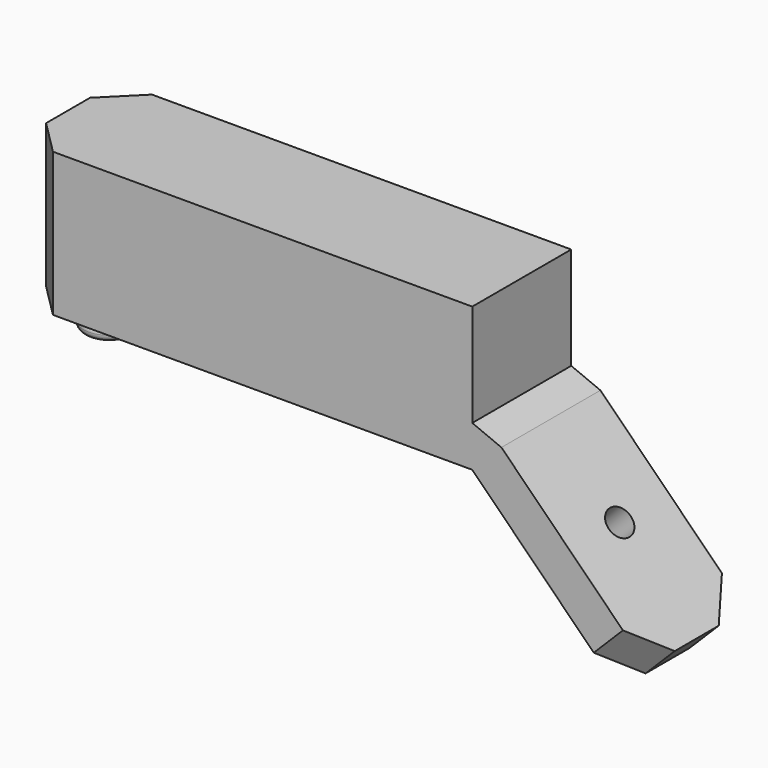
from build123d import *

# Parameters (mm, degrees)
F0_R      = 3.75
F1_DEPTH  = 2
F2_R      = 1
F3_DEPTH  = 3
F4_W      = 37.5
F4_H      = 18
F5_DEPTH  = 6
F7_DEPTH  = 18
F8_R      = 2
F9_DEPTH  = 37.8
F10_R     = 0.99999
F11_SIZE  = 5
F12_DEPTH = 14.9


# Not quite as in the source:
# - a fillet or chamfer is up to 0.001 mm smaller than in the source, because OpenCascade refuses the exact size


with BuildPart() as f1:
    # F0 (on Top) → F1 (new body)
    with BuildSketch(Plane.XY):
        Circle(F0_R)
    extrude(amount=F1_DEPTH)

    # F2 (on face) → F3 (join)
    with BuildSketch(Plane.XY.offset(2)):
        Circle(F2_R)
    extrude(amount=F3_DEPTH)

    # F4 (on face) → F5 (join)
    with BuildSketch(Plane.XY.offset(5)):
        with BuildLine():
            Line((22.5, 9), (0, 9))
            Line((0, 9), (0, 1))
            ThreePointArc((0, 1), (0.7071067812, 0.7071067812), (1, 0))
            ThreePointArc((1, 0), (0.7071067812, -0.7071067812), (0, -1))
            Line((0, -1), (0, -9))
            Line((0, -9), (22.5, -9))
            Line((22.5, -9), (22.5, 9))
        make_face()
        with BuildLine():
            ThreePointArc((1, 0), (0.7071067812, 0.7071067812), (0, 1))
            Line((0, 1), (0, -1))
            ThreePointArc((0, -1), (0.7071067812, -0.7071067812), (1, 0))
        make_face()
        with BuildLine():
            Line((0, -1), (0, 1))
            ThreePointArc((0, 1), (-1, 0), (0, -1))
        make_face()
        with BuildLine():
            Line((0, 9), (-6, 9))
            Line((-6, 9), (-6, -9))
            Line((-6, -9), (0, -9))
            Line((0, -9), (0, -1))
            ThreePointArc((0, -1), (-1, 0), (0, 1))
            Line((0, 1), (0, 9))
        make_face()
        with Locations((41.25, 0)):
            Rectangle(F4_W, F4_H)
    extrude(amount=F5_DEPTH)

    # F6 (on face) → F7 (join)
    with BuildSketch(Plane.XZ.offset(9)):
        Polygon((64.2426406871, 9.2426406871), (60, 5), (81.2132034356, -16.2132034356), (85.4558441227, -11.9705627485), align=None)
        Polygon((60, 11), (60, 5), (64.2426406871, 9.2426406871), align=None)
    extrude(amount=-F7_DEPTH)

    # F8 (on face) → F9 (cut)
    with BuildSketch(Plane(origin=(32.5, 0, 32.5), x_dir=(0, -1, 0), z_dir=(-0.7071067812, 0, -0.7071067812))):
        with Locations((0, -53.0515164137)):
            Circle(F8_R)
    extrude(amount=-F9_DEPTH, mode=Mode.SUBTRACT)

    # F10 (radius 1 in the source; OpenCascade refuses exactly that, so slightly less here)
    f10_edges = [f1.edges().sort_by_distance(p)[0] for p in [
        (-3.75, 0, 0),
        (-3.75, 0, 2),
    ]]
    fillet(f10_edges, radius=F10_R)

    # F11
    f11_edges = [f1.edges().sort_by_distance(p)[0] for p in [
        (-6, -9, 8),
        (-6, 9, 8),
        (83.334524, 9, -14.091883),
        (83.334524, -9, -14.091883),
    ]]
    chamfer(f11_edges, length=F11_SIZE)

    # F12 (add): a face of the model
    f12_faces = [f1.faces().sort_by_distance(p)[0] for p in [
        (27.6735454285, 0, 11),
    ]]
    extrude(f12_faces, amount=F12_DEPTH)


solid = f1.part
